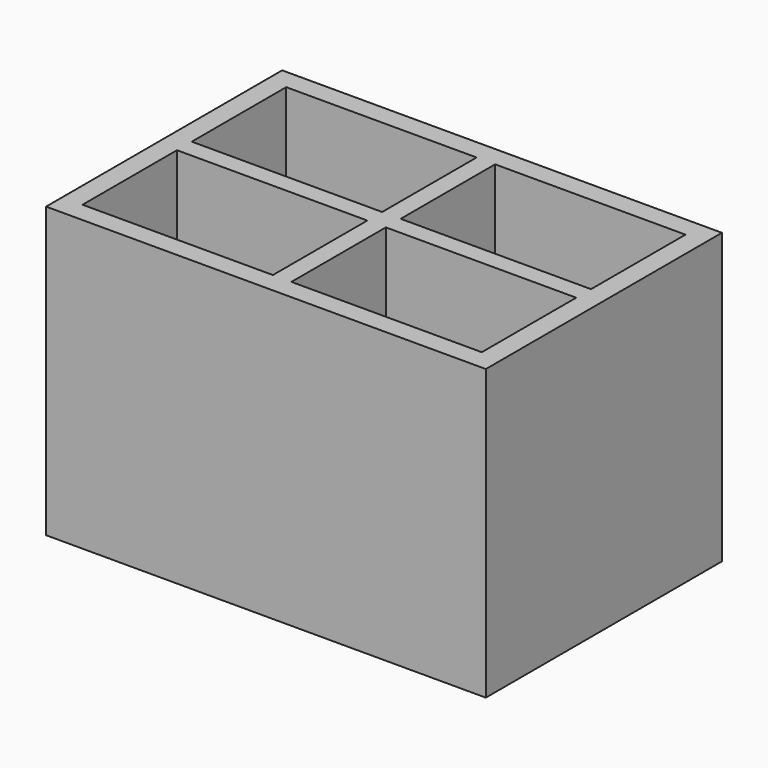
from build123d import *

# Parameters (mm, degrees)
F0_W     = 38
F0_H     = 25.5
F1_DEPTH = 25
F2_W     = 34.5
F2_H     = 22
F3_DEPTH = 20
F4_W     = 16.45
F4_H     = 1.6
F4_W_2   = 1.6
F4_H_2   = 10.2
F5_DEPTH = 20


with BuildPart() as f1:
    # F0 (on Top) → F1 (new body)
    with BuildSketch(Plane.XY):
        Rectangle(F0_W, F0_H)
    extrude(amount=F1_DEPTH)

    # F2 (on face) → F3 (cut)
    with BuildSketch(Plane.XY.offset(25)):
        Rectangle(F2_W, F2_H)
    extrude(amount=-F3_DEPTH, mode=Mode.SUBTRACT)

    # F4 (on face) → F5 (join)
    with BuildSketch(Plane.XY.offset(5)):
        with Locations((-9.025, 0)):
            Rectangle(F4_W, F4_H)
        with Locations((0, -5.9)):
            Rectangle(F4_W_2, F4_H_2)
        Rectangle(F4_W_2, F4_H)
        with Locations((0, 5.9)):
            Rectangle(F4_W_2, F4_H_2)
        with Locations((9.025, 0)):
            Rectangle(F4_W, F4_H)
    extrude(amount=F5_DEPTH)


solid = f1.part
